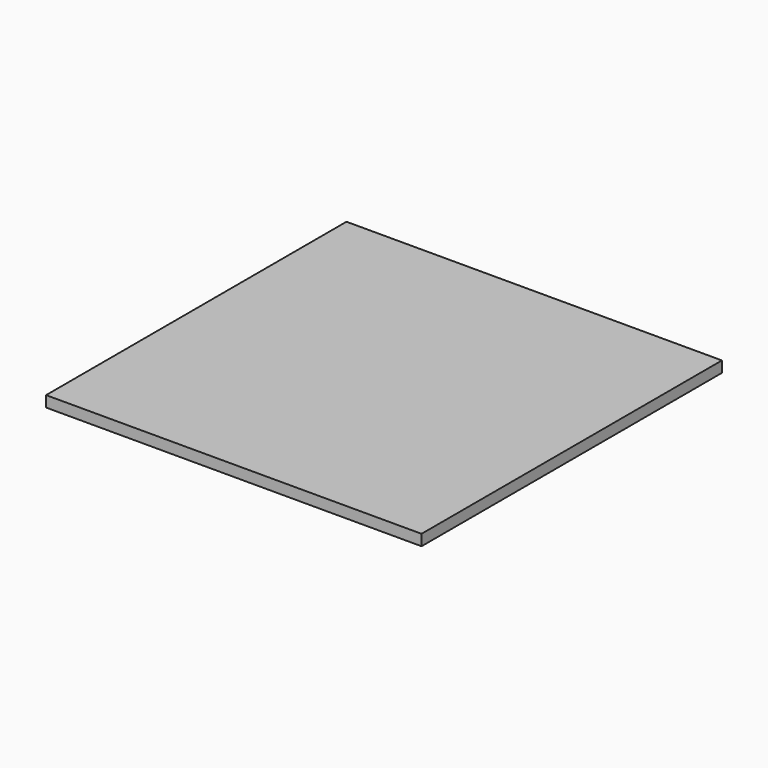
from build123d import *

# Parameters (mm, degrees)
F0_W     = 650
F0_H     = 650
F0_R     = 4
F1_DEPTH = 19
F2_DEPTH = 10


# Not quite as in the source:
# - a pattern or mirror of a feature is missing from the dataset's text; its kind, count and spacing are read off the source's solid


with BuildPart() as f1:
    # F0 (on Top) → F1 (new body)
    with BuildSketch(Plane.XY):
        Rectangle(F0_W, F0_H)
        with Locations((-315, -261)):
            Circle(F0_R, mode=Mode.SUBTRACT)
        with Locations((-315, -155.8)):
            Circle(F0_R, mode=Mode.SUBTRACT)
        with Locations((-315, -50.6)):
            Circle(F0_R, mode=Mode.SUBTRACT)
        with Locations((-315, 54.6)):
            Circle(F0_R, mode=Mode.SUBTRACT)
        with Locations((-315, 159.8)):
            Circle(F0_R, mode=Mode.SUBTRACT)
        with Locations((-315, 265)):
            Circle(F0_R, mode=Mode.SUBTRACT)
        with Locations((-315, 265)):
            Circle(F0_R)
        with Locations((-315, 159.8)):
            Circle(F0_R)
        with Locations((-315, 54.6)):
            Circle(F0_R)
        with Locations((-315, -50.6)):
            Circle(F0_R)
        with Locations((-315, -155.8)):
            Circle(F0_R)
        with Locations((-315, -261)):
            Circle(F0_R)
    extrude(amount=F1_DEPTH)

    # F0 (on Top) → F2 (cut)
    with BuildSketch(Plane.XY):
        with Locations((-315, 265)):
            Circle(F0_R)
        with Locations((-315, 159.8)):
            Circle(F0_R)
        with Locations((-315, 54.6)):
            Circle(F0_R)
        with Locations((-315, -50.6)):
            Circle(F0_R)
        with Locations((-315, -155.8)):
            Circle(F0_R)
        with Locations((-315, -261)):
            Circle(F0_R)
    f2 = extrude(amount=F2_DEPTH, mode=Mode.SUBTRACT)

    # F2_copies: F2 across plane
    add(f2.mirror(Plane(origin=(0, 0, 0), x_dir=(0, 0, 1), z_dir=(1, 0, 0))), mode=Mode.SUBTRACT)


solid = f1.part
